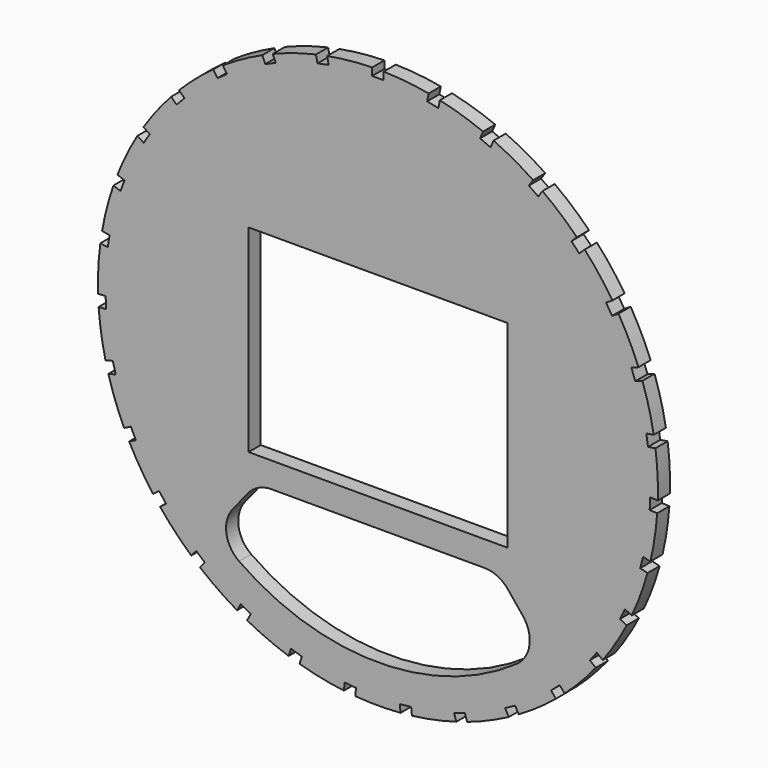
from build123d import *

# Parameters (mm, degrees)
F0_R     = 116.84
F0_W     = 107.95
F0_H     = 82.55
F1_DEPTH = 6.35
F3_DEPTH = 12.7


# Not quite as in the source:
# - ends of sketch curves that miss each other by under 0.0002 mm in the source are joined


with BuildPart() as f1:
    # F0 (on Front) → F1 (new body)
    with BuildSketch(Plane.XZ):
        Circle(F0_R)
        with BuildLine():
            ThreePointArc((57.9557025683, -82.6744686394), (0, -100.965), (-57.9557025683, -82.6744686394))
            ThreePointArc((-57.9557025683, -82.6744686394), (-63.2424676953, -74.0399131217), (-60.5362426444, -64.283798092))
            Line((-60.5362426444, -64.283798092), (-54.2551455528, -56.5256778711))
            ThreePointArc((-54.2551455528, -56.5256778711), (-49.8526531391, -53.0544887955), (-44.3845799964, -51.8170441872))
            Line((-44.3845799964, -51.8170441872), (44.3845799964, -51.8170441872))
            ThreePointArc((44.3845799964, -51.8170441872), (49.8526531391, -53.0544887955), (54.2551455528, -56.5256778711))
            Line((54.2551455528, -56.5256778711), (60.5362426444, -64.283798092))
            ThreePointArc((60.5362426444, -64.283798092), (63.2424676953, -74.0399131217), (57.9557025683, -82.6744686394))
        make_face(mode=Mode.SUBTRACT)
        Rectangle(F0_W, F0_H, mode=Mode.SUBTRACT)
    extrude(amount=F1_DEPTH)

    # F2 (on face) → F3 (cut, symmetric)
    with BuildSketch(Plane.XZ.offset(6.35)):
        Polygon((2.3792107569, 116.84), (-2.38125, 116.84), (-2.38125, 113.665), (2.3792661711, 113.665), align=None)
        Polygon((-2.38125, 113.665), (-2.38125, 116.84), (-2.3832892423, 116.8399584216), (-2.3832338281, 113.664958422), align=None)
        Polygon((2.38125, 116.84), (2.3792107569, 116.84), (2.3792661711, 113.6650415433), (2.38125, 113.665), align=None)
        Polygon((25.8521605942, 113.96895079), (21.1871487092, 114.9276323655), (20.5480276589, 111.8176244422), (25.2130395439, 110.8589428667), align=None)
        Polygon((48.2646865559, 106.4320251767), (43.8881478633, 108.3101400086), (42.6360713087, 105.3924475469), (47.0126100013, 103.514332715), align=None)
        Polygon((68.7012615192, 94.537784072), (64.7923710351, 97.2584423441), (62.9785988537, 94.6525153548), (66.8874893377, 91.9318570826), align=None)
        Polygon((86.3252143359, 78.7731764081), (83.0440016102, 82.2249946678), (80.742789437, 80.0375195173), (84.0240021628, 76.5857012576), align=None)
        Polygon((100.415022302, 59.7836035017), (97.8958198253, 63.8252646864), (95.2013790356, 62.1457963686), (97.7205815122, 58.1041351839), align=None)
        Polygon((110.3938502174, 38.3464963946), (108.7397938642, 42.8125353365), (105.7624345696, 41.709831101), (107.4164909228, 37.2437921591), align=None)
        Polygon((115.8531659566, 15.3394879114), (115.1319726134, 20.0470654638), (111.9935875785, 19.5662699016), (112.7147809217, 14.8586923493), align=None)
        Polygon((116.5694657294, -8.2955175322), (116.8106609728, -3.5391290804), (113.6397353383, -3.3783322514), (113.3985400948, -8.1347207032), align=None)
        Polygon((112.5134243011, -31.5909053937), (113.7071336244, -26.9804320664), (110.6334847395, -26.184625851), (109.4397754163, -30.7950991782), align=None)
        Polygon((103.8510955651, -53.5929650372), (105.9484486388, -49.3171591092), (103.0979113534, -47.9189237267), (101.0005582798, -52.1947296548), align=None)
        Polygon((90.9371143142, -73.4009345429), (93.8522457324, -69.6348470419), (91.3415207317, -67.6914260965), (88.4263893136, -71.4575135974), align=None)
        Polygon((74.3001775309, -90.2038778015), (77.9137421316, -87.1016919389), (75.8456182231, -84.6926488717), (72.2320536224, -87.7948347344), align=None)
        Polygon((54.6213995909, -103.3138841506), (58.7854584338, -101.0026030768), (57.2446043846, -98.2265638481), (53.0805455416, -100.537844922), align=None)
        Polygon((32.7064275147, -112.1942313615), (37.2505044854, -110.7684786712), (36.300002692, -107.7390940241), (31.7559257212, -109.1648467143), align=None)
        Polygon((9.4524578666, -116.4813589886), (14.1905189501, -115.9995048416), (13.869282852, -112.8407974526), (9.1312217685, -113.3226515996), align=None)
        Polygon((-14.1884943746, -115.9997524952), (-9.4504248819, -116.4815239474), (-9.1292439138, -113.3228109523), (-13.8673134065, -112.8410395), align=None)
        Polygon((-37.2485712051, -110.7691287983), (-32.704469351, -112.1948021792), (-31.7540204304, -109.1654009431), (-36.2981222845, -107.7397275622), align=None)
        Polygon((-58.7836955969, -101.0036290612), (-54.6195964151, -103.3148374582), (-53.0787908171, -100.538771337), (-57.2428899989, -98.22756294), align=None)
        Polygon((-77.9122219084, -87.1030517769), (-74.2986031649, -90.2051745705), (-72.2305213025, -87.7960954082), (-75.844140046, -84.6939726146), align=None)
        Polygon((-93.8510303607, -69.636485062), (-90.9358332124, -73.4025216837), (-88.4251421312, -71.4590569182), (-91.3403392796, -67.6930202964), align=None)
        Polygon((-105.9475878758, -49.3190082509), (-103.8501601756, -53.5947775726), (-100.9996472945, -52.1964924391), (-103.0970749947, -47.9207231174), align=None)
        Polygon((-113.7066627097, -26.9824166262), (-112.5128729187, -31.5928691186), (-109.4392379237, -30.797009258), (-110.6330277147, -26.1865567655), align=None)
        Polygon((-116.8105991856, -3.5411678105), (-116.5693209275, -8.2975520519), (-113.3983980999, -8.1366998799), (-113.639676358, -3.3803156385), align=None)
        Polygon((-115.1323224832, 20.0450560288), (-115.8534336636, 15.3374658899), (-112.7150402377, 14.856725103), (-111.9939290573, 19.5643152418), align=None)
        Polygon((-108.7405410673, 42.8106374625), (-110.3945194732, 38.3445696526), (-107.4171409332, 37.241917382), (-105.7631625274, 41.707985192), align=None)
        Polygon((-97.8969337715, 63.8235560723), (-100.4160657074, 59.7818509198), (-97.7215956058, 58.1024296292), (-95.2024636698, 62.1441347816), align=None)
        Polygon((-83.0454366945, 82.2235452641), (-86.3265891741, 78.7716697368), (-84.0253388226, 76.5842347504), (-80.744186343, 80.0361102776), align=None)
        Polygon((-64.7940685053, 97.2573114891), (-68.7029115043, 94.5365849944), (-66.8890938411, 91.9306896617), (-62.9802508421, 94.6514161565), align=None)
        Polygon((-43.8900382252, 108.3093739995), (-48.2665441378, 106.4311827828), (-47.0144166601, 103.5135121744), (-42.6379107474, 105.391703391), align=None)
        Polygon((-21.1891545716, 114.9272625625), (-25.8541497237, 113.9684995673), (-25.2149743936, 110.8585027993), (-20.5499792415, 111.8172657944), align=None)
    extrude(amount=F3_DEPTH, both=True, mode=Mode.SUBTRACT)


with BuildPart() as f4_1:
    # F4: copy of F1
    add(f1.part.moved(Location((0, 87.3125, 0))))


solid = f1.part
